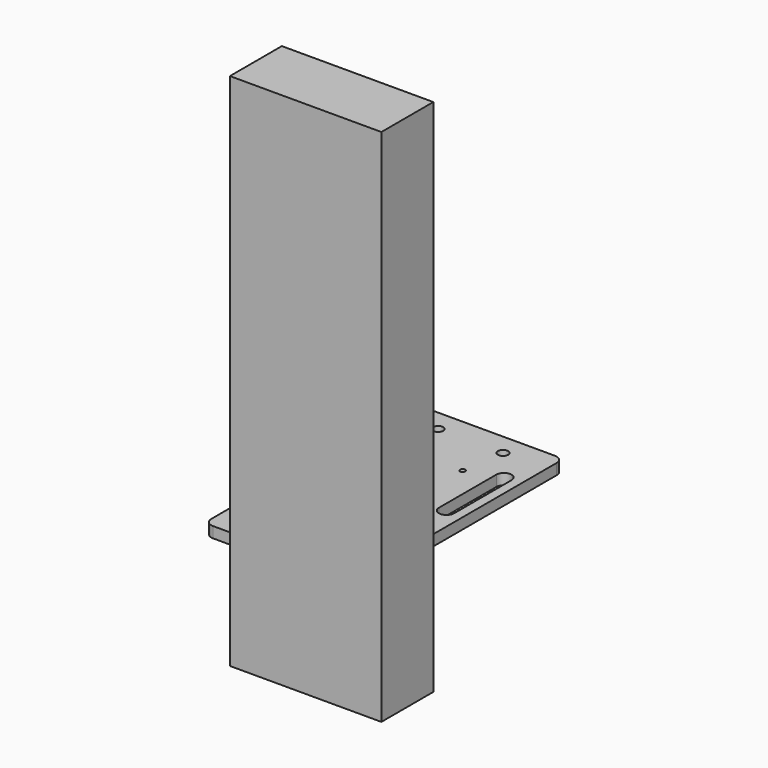
from build123d import *

# Parameters (mm, degrees)
F0_W     = 88.9
F0_H     = 152.4
F0_R     = 2.54
F0_R_2   = 1.5
F0_R_3   = 6.8073941992
F0_R_4   = 3
F1_DEPTH = 6.35
F2_R     = 5.08
F3_W     = 88.9
F3_H     = 38.1
F4_DEPTH = 304.8


# Not quite as in the source:
# - a length typed as a fraction of an inch, garbled in the dataset ("3 / 203.2 mm" for 3/8 in), is restored


with BuildPart() as f1:
    # F0 (on Top) → F1 (new body)
    with BuildSketch(Plane.XY):
        with Locations((-122.368119657, 209.6838048907)):
            Rectangle(F0_W, F0_H)
        with Locations((-151.9854813814, 144.194945693)):
            Circle(F0_R, mode=Mode.SUBTRACT)
        with Locations((-122.368119657, 160.7289016247)):
            Circle(F0_R, mode=Mode.SUBTRACT)
        with Locations((-92.7507579327, 144.194945693)):
            Circle(F0_R, mode=Mode.SUBTRACT)
        with BuildLine():
            Line((-161.3446665764, 212.3949378729), (-161.3446665764, 254.4926702976))
            ThreePointArc((-161.3446665764, 254.4926702976), (-156.8996665764, 258.9376702976), (-152.4546665764, 254.4926702976))
            Line((-152.4546665764, 254.4926702976), (-152.4546665764, 212.3949378729))
            ThreePointArc((-152.4546665764, 212.3949378729), (-156.8996665764, 207.9499378729), (-161.3446665764, 212.3949378729))
        make_face(mode=Mode.SUBTRACT)
        with Locations((-137.868119657, 216.9896082271)):
            Circle(F0_R_2, mode=Mode.SUBTRACT)
        with Locations((-122.368119657, 232.4896082271)):
            Circle(F0_R_3, mode=Mode.SUBTRACT)
        with Locations((-137.868119657, 247.9896082271)):
            Circle(F0_R_2, mode=Mode.SUBTRACT)
        with Locations((-141.418119657, 273.1838048907)):
            Circle(F0_R_4, mode=Mode.SUBTRACT)
        with Locations((-106.868119657, 216.9896082271)):
            Circle(F0_R_2, mode=Mode.SUBTRACT)
        with BuildLine():
            Line((-92.2815727377, 212.3949378729), (-92.2815727377, 254.4926702976))
            ThreePointArc((-92.2815727377, 254.4926702976), (-87.8365727377, 258.9376702976), (-83.3915727377, 254.4926702976))
            Line((-83.3915727377, 254.4926702976), (-83.3915727377, 212.3949378729))
            ThreePointArc((-83.3915727377, 212.3949378729), (-87.8365727377, 207.9499378729), (-92.2815727377, 212.3949378729))
        make_face(mode=Mode.SUBTRACT)
        with Locations((-106.868119657, 247.9896082271)):
            Circle(F0_R_2, mode=Mode.SUBTRACT)
        with Locations((-103.318119657, 273.1838048907)):
            Circle(F0_R_4, mode=Mode.SUBTRACT)
    extrude(amount=F1_DEPTH)

    # F2
    f2_edges = [f1.edges().sort_by_distance(p)[0] for p in [
        (-77.91812, 285.883805, 3.175),
        (-166.81812, 285.883805, 3.175),
        (-77.91812, 133.483805, 3.175),
        (-166.81812, 133.483805, 3.175),
    ]]
    fillet(f2_edges, radius=F2_R)


with BuildPart() as f4:
    # F3 (on Top) → F4 (new body)
    with BuildSketch(Plane.XY):
        with Locations((-32.1518591821, 58.4733763218)):
            Rectangle(F3_W, F3_H)
    extrude(amount=F4_DEPTH)


solid = Compound([f1.part, f4.part])
